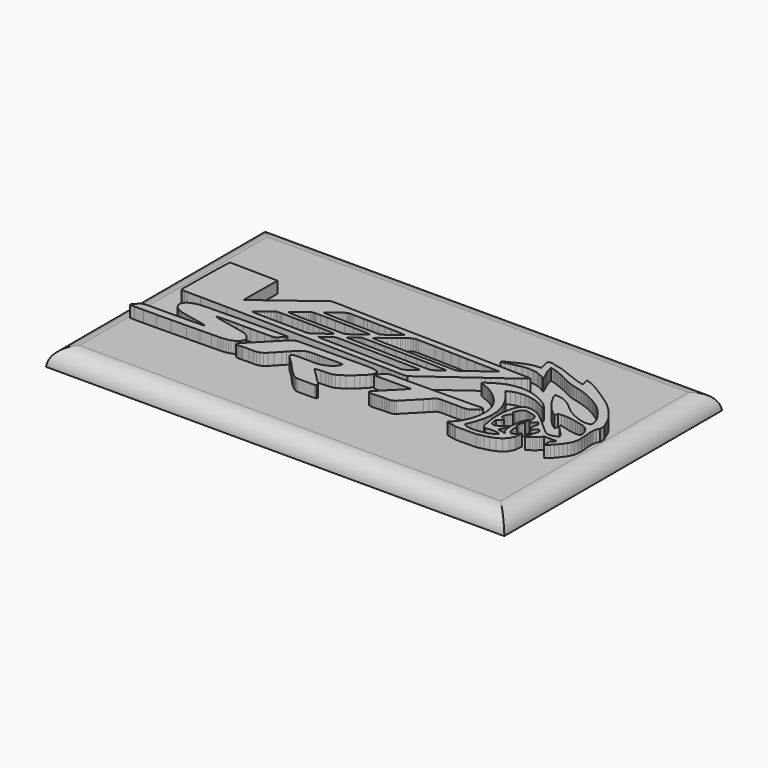
from build123d import *

# Parameters (mm, degrees)
F0_W        = 125.6636679173
F0_H        = 74.59346205
F1_DEPTH    = 4.7625
F3_DEPTH    = 3.175
F4_T1_DEPTH = 151.0140100007
F4_T3_DEPTH = 99.9438041335


# Not quite as in the source:
# - a fillet or chamfer that OpenCascade refuses, or shapes differently, is made with other operations: its cross-section is extruded or revolved along the edge and cut away or added


with BuildPart() as f1:
    # F0 (on Top) → F1 (new body)
    with BuildSketch(Plane.XY):
        Rectangle(F0_W, F0_H)
    extrude(amount=F1_DEPTH)

    # F2 (on face) → F3 (join)
    with BuildSketch(Plane.XY.offset(4.7625)):
        Polygon((-4.9450498, -8.5601048), (-4.421759, -8.639302), (-4.5465492, -9.1872054), (-4.8525684, -9.7208086), (-5.3076602, -10.224897), (-5.8802524, -10.6841036), (-6.5382648, -11.0831122), (-7.2498712, -11.4066066), (-7.9832708, -11.6391944), (-8.7064596, -11.7656102), (-9.5160592, -11.8009924), (-10.570972, -11.7964966), (-11.7620542, -11.7747034), (-12.9804668, -11.7577108), (-14.1171676, -11.7679978), (-15.0630636, -11.8277894), (-15.7091634, -11.95959), (-15.9465518, -12.1857008), (-15.8717742, -12.453112), (-15.6735526, -12.76731), (-15.3829512, -13.113512), (-15.0311612, -13.476605), (-14.2674594, -14.193901), (-13.6305544, -14.7994116), (-13.1164584, -15.3579068), (-12.4780548, -16.0731962), (-11.7503702, -16.876903), (-10.968355, -17.700498), (-10.1670612, -18.4758076), (-9.3814646, -19.134201), (-8.6465664, -19.6075046), (-7.9972662, -19.8271892), (-3.2755586, -19.8046086), (-2.797556, -19.6833998), (-2.6407618, -19.4626992), (-2.745867, -19.1551052), (-3.053461, -18.773394), (-3.504057, -18.330291), (-4.0383714, -17.8386994), (-4.5968666, -17.3112938), (-5.120259, -16.760698), (-5.4525672, -16.3987988), (-5.8057542, -16.0437068), (-6.1711586, -15.6935932), (-6.539865, -15.3470102), (-6.9028564, -15.0022052), (-7.2514714, -14.6572986), (-7.5766676, -14.3107918), (-7.869555, -13.9610084), (-6.2843664, -13.790803), (-5.0888646, -13.7265918), (-4.1617646, -13.6871964), (-3.381756, -13.5911082), (-2.6275538, -13.3571996), (-1.7779492, -12.9041906), (-0.711454, -12.1509028), (0.6931406, -11.0159038), (1.6305276, -10.2006908), (2.5060402, -9.348597), (3.211449, -8.5052916), (3.6384484, -7.716901), (3.6787328, -7.0292976), (3.2240474, -6.4884046), (2.1661374, -6.140196), (0.3966464, -6.030595), (-16.7135556, -6.2076076), (-17.6600612, -6.2193932), (-18.3821578, -6.2480952), (-18.9333632, -6.3112904), (-19.3670682, -6.4268096), (-19.7366636, -6.612509), (-20.0956672, -6.8859908), (-20.4974698, -7.265289), (-20.9954622, -7.7680058), (-28.045664, -14.961108), (-28.1941524, -15.2684988), (-28.1600656, -15.4747976), (-27.9811734, -15.5981908), (-27.6953726, -15.657195), (-27.3407632, -15.6701998), (-26.9550642, -15.6555948), (-26.576274, -15.6316934), (-26.242264, -15.6170122), (-24.5495572, -15.6137102), (-23.3030522, -15.6145992), (-22.3775524, -15.5568904), (-21.6474548, -15.3779982), (-20.9874612, -15.0153116), (-20.2721718, -14.4058894), (-19.3761614, -13.4872984), (-18.1740556, -12.196699), (-17.5040544, -11.4781076), (-16.752062, -10.6875072), (-16.366871, -10.2960932), (-15.98676, -9.923907), (-15.6206698, -9.5829882), (-15.2768554, -9.2860114), (-14.7908518, -8.9778078), (-14.2279624, -8.768207), (-13.6040622, -8.639302), (-12.9347722, -8.573008), (-12.2358658, -8.551291), (-11.5231672, -8.5560916), (-10.8124498, -8.5694012), (-10.1194616, -8.5732112), (-9.5076518, -8.5608922), (-8.7845646, -8.5400896), (-7.9914496, -8.5179916), (-7.1695564, -8.5017102), (-6.3603632, -8.4984082), (-5.6050688, -8.5155024), align=None)
        Polygon((-56.7795664, -14.6026886), (-57.280556, -14.9388068), (-57.2752728, -15.4519122), (-56.0680616, -15.5184094), (-53.5015694, -15.5360116), (-49.9995698, -15.516606), (-45.9858618, -15.4722068), (-41.8842698, -15.4148028), (-38.1184658, -15.3565098), (-35.1122742, -15.3092912), (-33.2894686, -15.285212), (-32.6026526, -15.2675082), (-31.9255648, -15.2214072), (-31.2669682, -15.1413972), (-30.6357528, -15.0217886), (-30.040453, -14.8571966), (-29.4899588, -14.6420078), (-28.9930586, -14.3704056), (-28.558363, -14.0370052), (-28.1099514, -13.4955026), (-27.9135586, -12.9533904), (-27.931872, -12.4250958), (-28.12796, -11.9251984), (-28.4644592, -11.4683032), (-28.9043618, -11.068812), (-29.4103552, -10.7412028), (-29.945457, -10.5002076), (-30.9034688, -10.21969), (-32.2077588, -9.9157028), (-33.7221576, -9.5976948), (-35.310572, -9.2750132), (-36.836858, -8.9571068), (-38.1648716, -8.6536022), (-39.1583672, -8.3737958), (-39.6813532, -8.127111), (-37.7867672, -8.075295), (-35.8783636, -8.0485996), (-33.962467, -8.0388968), (-32.0455544, -8.0381094), (-30.134052, -8.0383888), (-28.2345638, -8.0315054), (-26.353262, -8.0096106), (-24.4967506, -7.9645002), (-24.1630708, -7.9471012), (-23.8976662, -7.916291), (-23.684357, -7.8685898), (-23.5072682, -7.8001114), (-23.3501692, -7.7071982), (-23.197058, -7.5861926), (-23.0320596, -7.4332084), (-22.8389688, -7.244588), (-22.525863, -6.9569076), (-22.1765622, -6.6300096), (-22.0138498, -6.4578992), (-21.8727528, -6.2830964), (-21.7635582, -6.1080904), (-21.6963498, -5.9352942), (-22.897973, -5.86359), (-25.3242572, -5.8418984), (-28.5935674, -5.8582052), (-32.3243702, -5.900293), (-36.1351576, -5.9560968), (-39.6444724, -6.0136024), (-42.4707558, -6.0605924), (-44.2323728, -6.0851034), (-46.042961, -6.2347094), (-47.4401642, -6.6143124), (-48.4317548, -7.1706994), (-49.0252512, -7.8509114), (-49.2283496, -8.60171), (-49.0487716, -9.369806), (-48.494061, -10.1022912), (-47.5718632, -10.7459018), (-47.0938606, -10.9669072), (-46.5738718, -11.1561118), (-46.02226, -11.3192052), (-45.4497694, -11.462004), (-44.8667632, -11.5901978), (-44.2839602, -11.7096032), (-43.711749, -11.8259098), (-43.1608738, -11.9449088), (-42.8145702, -12.016613), (-42.2718738, -12.123801), (-41.6006534, -12.258294), (-40.8686508, -12.4122942), (-40.1436586, -12.5778006), (-39.4932662, -12.7468884), (-38.9852662, -12.9116074), (-38.6874512, -13.0640074), (-39.391463, -13.1373118), (-40.9285694, -13.1928108), (-43.0484534, -13.2329936), (-45.5008742, -13.260705), (-48.0355656, -13.2786882), (-50.4022614, -13.2896102), (-52.3507716, -13.2961888), (-53.6307538, -13.3012942), (-54.6571678, -13.339191), (-55.3450506, -13.4348982), (-55.7820576, -13.5832088), (-56.056149, -13.7791952), (-56.2552596, -14.0178028), (-56.4670702, -14.2940024), align=None)
        Polygon((4.0287448, -8.0929988), (3.9759382, -8.375396), (13.9917424, -8.3471004), (13.730732, -8.708009), (13.242036, -9.2605098), (12.59205, -9.946005), (11.8471442, -10.7063032), (11.0737396, -11.4830098), (10.3381302, -12.2177048), (9.7068386, -12.8520952), (9.246235, -13.3277102), (8.6214458, -13.947013), (8.1675478, -14.3867124), (8.0184498, -14.5703036), (7.928737, -14.7463002), (7.903845, -14.927199), (7.9493364, -15.1253952), (8.3251294, -15.2392888), (8.7700358, -15.3008076), (9.2644468, -15.3212038), (9.7887282, -15.3118058), (10.3231442, -15.2838912), (10.8479336, -15.2487884), (11.34364, -15.2178004), (11.7905276, -15.2021032), (12.3123452, -15.2064974), (12.8007364, -15.219807), (13.2577332, -15.2258014), (13.6855454, -15.2078944), (14.0862304, -15.1499062), (14.461744, -15.035403), (14.8141436, -14.8481034), (15.145639, -14.571599), (19.1523366, -10.4836976), (20.0035414, -9.5811086), (20.5969362, -8.9512902), (21.0416394, -8.546592), (21.4469472, -8.3194906), (21.9220288, -8.2222086), (22.5761296, -8.206994), (23.5185458, -8.2263996), (24.8582434, -8.2325972), (26.4908284, -8.2333084), (27.713051, -8.2496914), (28.6145478, -8.245602), (29.285438, -8.1849976), (29.815536, -8.0315054), (30.2947324, -7.7491082), (30.8129432, -7.3015094), (31.4601352, -6.6525902), (31.8035432, -6.2350904), (31.8998346, -5.953506), (31.789751, -5.7833006), (31.514034, -5.6999886), (31.113349, -5.6791098), (30.6284376, -5.6961024), (30.1000414, -5.7264046), (29.5689274, -5.7457086), (9.5561404, -5.952109), (9.1602306, -5.9466988), (8.6710266, -5.9301126), (8.1235296, -5.9117992), (7.5532488, -5.9015884), (6.9952362, -5.9090052), (6.484747, -5.9436), (6.0570364, -6.015101), (5.7473342, -6.1331094), (5.6303418, -6.2255908), (5.4055264, -6.4247014), (5.1118262, -6.7041014), (4.7882302, -7.0370954), (4.4739306, -7.3972928), (4.2077386, -7.7580998), align=None)
        Polygon((30.560137, 10.9086904), (31.0405272, 11.3337086), (30.5953414, 11.4064034), (30.0228508, 11.457305), (29.3624508, 11.4908076), (28.6534352, 11.5112038), (27.9352502, 11.5229894), (27.2471388, 11.5305078), (26.6284456, 11.538204), (26.1185406, 11.5502944), (20.4317346, 11.729212), (14.707743, 11.868912), (8.9595452, 11.9830088), (3.1997396, 12.0850914), (-2.5587706, 12.1885964), (-8.3031584, 12.307189), (-14.020673, 12.4544074), (-19.698462, 12.6437898), (-20.1191622, 12.6592076), (-20.7461612, 12.6799086), (-21.5059514, 12.7007874), (-22.324949, 12.7169926), (-23.129367, 12.7235966), (-23.8456724, 12.715494), (-24.4001544, 12.687808), (-24.719153, 12.6355094), (-36.6615726, 3.6841938), (-38.1194564, 2.590292), (-38.4727704, 2.3146004), (-38.8779512, 1.992503), (-39.089457, 1.843405), (-39.3012676, 1.7179036), (-39.5091666, 1.6279114), (-39.708963, 1.5849092), (-39.5792706, 12.9772918), (-52.8131532, 13.2104892), (-52.8919694, 11.9055896), (-52.9518626, 10.2175056), (-52.9962618, 8.2658966), (-53.0283674, 6.170803), (-53.0515576, 4.0520112), (-53.0691598, 2.0294092), (-53.0844506, 0.2227072), (-53.100859, -1.2480036), (-53.1241508, -1.9560032), (-53.148357, -2.4705056), (-53.1395686, -2.822194), (-53.0638512, -3.0420056), (-52.8874736, -3.1606998), (-52.5764506, -3.208909), (-52.0969494, -3.2174942), (-51.4152642, -3.2171894), (-47.769653, -3.2425894), (-40.5159718, -3.3504124), (2.7827478, -4.1852088), (3.3846262, -4.2026078), (4.2793412, -4.2317924), (5.3608478, -4.2646092), (6.523228, -4.2928032), (7.6607416, -4.3081956), (8.6674452, -4.3027092), (9.4374462, -4.2681906), (9.8648266, -4.1963086), (22.663531, 5.1201066), (23.2379266, 5.531104), (24.2443508, 6.2514988), (25.5343406, 7.1790052), (26.959433, 8.2109056), (28.371038, 9.2447872), (29.620845, 10.178288), align=None)
        Polygon((-33.6645504, -1.7394936), (-34.9256604, -1.6497046), (-34.7867732, -1.4484096), (-34.4552524, -1.1359896), (-33.9890608, -0.7499096), (-33.4457548, -0.3271012), (-32.8831702, 0.0950976), (-32.358965, 0.4796028), (-31.9308734, 0.7892034), (-31.656655, 0.9866884), (-31.3305698, 1.2276074), (-31.085155, 1.4076934), (-30.8845712, 1.5357094), (-30.6929536, 1.620393), (-30.4744628, 1.6705072), (-30.1931578, 1.6948912), (-29.8131738, 1.702308), (-29.2986714, 1.7013936), (-26.3820656, 1.6632936), (-24.9446542, 1.640205), (-23.48865, 1.6244062), (-22.0210634, 1.610487), (-20.5483714, 1.5930118), (-19.0774574, 1.5664942), (-17.6150524, 1.525397), (-16.167862, 1.4642084), (-14.742668, 1.3775944), (-14.8617686, 1.2030964), (-15.0341584, 1.0205974), (-15.2450546, 0.8349996), (-15.4795728, 0.651002), (-15.959963, 0.3070098), (-16.3567618, 0.0270002), (-17.125569, -0.564388), (-17.7068734, -1.0321036), (-18.1571646, -1.388999), (-18.5332624, -1.6480028), (-18.8916564, -1.8218912), (-19.2890648, -1.9235928), (-19.782155, -1.9660108), (-20.4274674, -1.961896), (-21.963761, -1.9281902), (-23.815167, -1.9059906), (-25.8636516, -1.8886932), (-27.991054, -1.8699988), (-30.079061, -1.8432018), (-32.0096642, -1.8019014), align=None, mode=Mode.SUBTRACT)
        Polygon((-16.2069526, -1.9470116), (-16.446754, -1.8266918), (-15.8980632, -1.4556994), (-15.4226514, -1.0815066), (-14.99235, -0.7209028), (-14.5788634, -0.3904996), (-14.1540738, -0.1070102), (-13.689457, 0.1131062), (-13.157073, 0.2530094), (-12.5284738, 0.2960116), (10.0730304, -0.201295), (9.9530408, -0.3319018), (9.6614488, -0.604393), (9.2428314, -0.9705086), (8.7416386, -1.3818108), (8.202549, -1.7899126), (7.6699364, -2.1463), (7.1885302, -2.4026114), (6.8028312, -2.5105106), (6.3747396, -2.5166066), (5.897245, -2.5015952), (5.4142386, -2.4790908), (4.970145, -2.4625046), (-9.3823536, -2.1745956), (-13.0148584, -2.0992084), (-13.3876542, -2.0981924), (-13.8466576, -2.1028914), (-14.3567658, -2.1058124), (-14.8828506, -2.0992084), (-15.3899616, -2.0756118), (-15.8429706, -2.0274026), align=None, mode=Mode.SUBTRACT)
        Polygon((-27.8380698, 2.9001974), (-28.6586676, 3.009011), (-28.4420564, 3.288411), (-28.0859738, 3.628898), (-27.6302724, 4.0091106), (-27.1145508, 4.4076112), (-26.5787632, 4.8032924), (-26.062559, 5.1747928), (-25.6055622, 5.5007002), (-25.2476508, 5.759704), (-25.031065, 5.9200034), (-24.8581672, 6.0411868), (-24.708358, 6.1287914), (-24.561165, 6.188202), (-24.3959634, 6.224905), (-24.192357, 6.2443868), (-23.9296702, 6.2521084), (-23.5873544, 6.2534038), (-22.4404682, 6.2504066), (-20.5767686, 6.23951), (-18.2504588, 6.218301), (-15.7157674, 6.1842904), (-13.2267706, 6.1348112), (-11.0377732, 6.0673996), (-9.4027498, 5.9794902), (-8.5759544, 5.8685938), (-8.757158, 5.6912002), (-8.9485724, 5.5221886), (-9.1484704, 5.3598064), (-9.3551502, 5.2020978), (-9.7821496, 4.892802), (-10.2160578, 4.5793914), (-10.9113574, 4.047998), (-11.4582702, 3.612388), (-11.9033544, 3.265805), (-12.2930666, 3.0012894), (-12.6740666, 2.8120086), (-13.0928618, 2.6907998), (-13.595858, 2.6310082), (-14.2298674, 2.6254964), (-15.6094684, 2.6502106), (-17.5122586, 2.67081), (-19.7371716, 2.6926032), (-22.0831664, 2.721102), (-24.3492528, 2.7615896), (-26.3345676, 2.8195016), align=None, mode=Mode.SUBTRACT)
        Polygon((-21.166963, 7.4673968), (-22.5784664, 7.5470004), (-22.4086674, 7.7727048), (-22.072473, 8.086598), (-21.6188544, 8.4589112), (-21.0971638, 8.8597994), (-20.5562708, 9.2594938), (-20.045553, 9.6280986), (-19.6140578, 9.9357942), (-19.3109596, 10.1528118), (-18.9929516, 10.3791004), (-18.737453, 10.5426002), (-18.5156602, 10.6527092), (-18.2988712, 10.7189016), (-18.0580538, 10.7506008), (-17.7644552, 10.7572048), (-17.3892718, 10.7481878), (-16.903573, 10.7329986), (-14.109065, 10.6643932), (-13.097764, 10.6466894), (-11.6615718, 10.6258106), (-9.9529646, 10.5999026), (-8.1238598, 10.5671874), (-6.3266574, 10.5259886), (-4.7135542, 10.4745028), (-3.4367724, 10.4109012), (-2.648458, 10.3335074), (-2.7795728, 10.1570028), (-3.1052516, 9.8624898), (-3.5671506, 9.4886018), (-4.1071546, 9.073896), (-4.666869, 8.6570058), (-5.18795, 8.2767932), (-5.6121554, 7.97179), (-5.8812684, 7.7806042), (-6.228969, 7.5359006), (-6.4874648, 7.3648062), (-6.6944494, 7.2554084), (-6.8875656, 7.1954898), (-7.1045578, 7.1732902), (-7.3830688, 7.1764906), (-7.7608684, 7.1933054), (-8.275574, 7.2115934), (-11.1920528, 7.2487028), (-12.6103634, 7.2760078), (-14.0348716, 7.296912), (-15.463266, 7.3159874), (-16.8930574, 7.3380092), (-18.3218582, 7.3674986), (-19.7472554, 7.4091038), align=None, mode=Mode.SUBTRACT)
        Polygon((-8.7423498, 1.5164054), (-11.5343686, 1.5914878), (-11.4738658, 1.7419066), (-11.4031522, 1.844294), (-11.2963706, 1.943989), (-11.1276638, 2.0862036), (-10.6380534, 2.450592), (-10.1958648, 2.7770074), (-9.8806508, 3.040888), (-9.6477582, 3.2476948), (-9.4526608, 3.402711), (-9.250553, 3.5113976), (-8.9968578, 3.5790886), (-8.647049, 3.6113974), (-8.1564734, 3.6135056), (-5.3978556, 3.5666934), (-2.5350724, 3.5265106), (0.3919474, 3.4869882), (3.343529, 3.4424112), (6.2798452, 3.3869884), (9.1608402, 3.3149032), (11.9469408, 3.220212), (14.5982436, 3.0973014), (14.46784, 2.9187902), (14.2046452, 2.6480008), (13.834745, 2.3208996), (13.3838442, 1.973199), (12.877927, 1.6407892), (12.3429268, 1.359408), (11.8047262, 1.1648948), (11.2891316, 1.093089), (8.5328506, 1.1131042), (5.703951, 1.1535918), (2.8248356, 1.2104116), (-0.0818642, 1.2792964), (-2.9935678, 1.356106), (-5.887974, 1.436497), align=None, mode=Mode.SUBTRACT)
        Polygon((-6.0683648, 4.7966884), (-7.1581518, 4.866894), (-6.9075554, 5.166487), (-6.3484506, 5.6504078), (-5.5785512, 6.2552072), (-4.695952, 6.91769), (-3.79857, 7.5747118), (-2.9842714, 8.1626964), (-2.3509732, 8.6187026), (-1.9966686, 8.879205), (-1.4768576, 9.2888054), (-1.0537698, 9.6216978), (-0.6962648, 9.8838004), (-0.3729736, 10.0812092), (-0.0526542, 10.2198932), (0.2958338, 10.3059992), (0.703834, 10.345293), (1.2026392, 10.3439976), (5.8098436, 10.2296976), (8.0340454, 10.1691948), (10.2696264, 10.1009958), (12.512548, 10.0293932), (14.7587462, 9.9586034), (17.0042332, 9.8929952), (19.244945, 9.836912), (21.4767414, 9.7943924), (23.6956346, 9.7700084), (23.5504482, 9.5602044), (23.2856278, 9.3020896), (22.9365302, 9.01319), (22.5382328, 8.7111078), (21.734526, 8.1372964), (21.1558378, 7.721092), (20.476845, 7.2081898), (19.816826, 6.7336924), (19.1565276, 6.2676024), (18.4769506, 5.779897), (17.93875, 5.3738018), (17.518634, 5.0435002), (17.177639, 4.7833026), (16.8769284, 4.5870876), (16.5777418, 4.449191), (16.2410394, 4.3636946), (15.8280354, 4.324604), (15.2998424, 4.3262042), (1.81483, 4.6383956), (0.7114286, 4.6602904), (-0.4115562, 4.6742096), (-1.5467584, 4.684903), (-2.6872692, 4.6975014), (-3.8257734, 4.716907), (-4.955159, 4.7483014), align=None, mode=Mode.SUBTRACT)
        Polygon((32.380047, -16.0050988), (32.5152258, -16.0567116), (38.3087372, -15.9968946), (38.9413496, -15.798292), (39.9464276, -15.5827984), (41.1772354, -15.2748996), (42.4866308, -14.7992084), (43.7278272, -14.080109), (44.7537332, -13.0421126), (45.4175368, -11.6099082), (45.5721466, -9.7079054), (45.3336406, -9.858502), (45.1495414, -10.0535994), (44.9928488, -10.2733094), (44.836334, -10.4974898), (44.6528444, -10.7061), (44.415329, -10.8789978), (44.0965336, -10.9961934), (43.669331, -11.0375954), (43.3635404, -10.7725972), (43.1206402, -10.4801924), (42.9409352, -10.1603048), (42.825035, -9.81329), (42.7732444, -9.4393004), (42.7859444, -9.0384122), (42.863643, -8.6107016), (43.0067466, -8.1564988), (42.5176442, -7.7380084), (42.394251, -7.4679048), (42.3420286, -7.1595996), (42.3526458, -6.8301108), (42.4176444, -6.4965072), (42.528744, -6.1762132), (42.6776388, -5.886196), (42.8558452, -5.6438038), (43.0552352, -5.4660038), (42.9651414, -5.3001926), (42.8605442, -5.1416966), (42.8132494, -5.0510948), (42.7749462, -4.9452022), (42.7497494, -4.818507), (42.74185, -4.665091), (42.7694344, -4.4936918), (42.8285402, -4.3035982), (42.8900336, -4.0799004), (42.92473, -3.8074092), (42.4467274, -4.3829986), (42.0885366, -5.0809906), (41.8371274, -5.87121), (41.6794442, -6.7233038), (41.6024314, -7.6070968), (41.5930334, -8.4923122), (41.6382454, -9.3486986), (41.7250372, -10.1460046), (41.7805362, -10.4851962), (41.8460428, -10.7548934), (41.9248336, -10.971403), (42.0203376, -11.1508032), (42.1360346, -11.3094008), (42.2751504, -11.4632994), (42.4411394, -11.6287042), (42.6374306, -11.821795), (40.4531322, -11.4625882), (40.541829, -11.0999016), (40.692451, -10.783189), (40.8776424, -10.491089), (41.069641, -10.2023926), (41.2411418, -9.8956114), (41.364535, -9.5496126), (41.4122362, -9.1429078), (41.3567372, -8.6542118), (40.6959308, -9.1988894), (40.0021298, -9.712706), (39.3145264, -10.1269038), (38.6724398, -10.3726996), (38.1150368, -10.3813102), (37.6814334, -10.0840032), (37.4109488, -9.4119954), (37.3426482, -8.2965036), (37.7731274, -7.9920084), (38.1262382, -7.7346048), (38.2745488, -7.6056998), (38.404546, -7.467092), (38.516433, -7.3116948), (38.6106416, -7.1322946), (38.4561334, -7.0092062), (38.3047494, -6.906895), (38.1553466, -6.8188078), (38.0066296, -6.7383914), (37.706935, -6.5746122), (37.3959374, -6.3631064), (37.3745506, -5.9075066), (37.4319292, -5.5110126), (37.5530364, -5.1656996), (37.7222258, -4.8633888), (37.924232, -4.5962062), (38.1437388, -4.3558968), (38.3652268, -4.134612), (38.573329, -3.9241984), (38.4922268, -3.7995098), (38.424231, -3.713099), (38.362636, -3.652901), (38.3007362, -3.6068), (38.1489458, -3.5081972), (37.9149356, -3.3198054), (37.948235, -3.078099), (38.0165356, -2.8228036), (38.1130302, -2.5614884), (38.230937, -2.3015956), (38.3633472, -2.0505928), (38.5034282, -1.8162016), (38.644449, -1.6056102), (38.77945, -1.426591), (38.9928354, -1.2187936), (39.237031, -1.0772902), (39.5079474, -0.993394), (39.8017492, -0.9582912), (40.1145502, -0.963295), (40.4422356, -0.9995916), (40.7810462, -1.0584942), (41.1269434, -1.131189), (42.0337488, -1.3830046), (42.6194474, -1.6639032), (42.9564292, -1.9832066), (43.1172366, -2.3499064), (43.1744374, -2.7734006), (43.200447, -3.2629094), (43.2677316, -3.8276022), (43.4488336, -4.4766992), (43.6525416, -4.4653962), (43.840146, -4.4392088), (44.0125358, -4.3967908), (44.170727, -4.336796), (44.3159388, -4.2575988), (44.4489332, -4.1579038), (44.5709294, -4.0362886), (44.6828418, -3.8913054), (44.7373502, -3.7960046), (44.9654422, -3.3866074), (45.2382382, -3.6563046), (45.5012298, -3.9067994), (45.6059286, -4.0402002), (45.68063, -4.1870122), (45.7161392, -4.3534076), (45.7030328, -4.5455078), (45.659929, -4.6908974), (45.6094338, -4.7706026), (45.556932, -4.8283114), (45.5081386, -4.9077118), (45.4682352, -5.0523902), (45.4430384, -5.3062124), (45.437933, -5.7126124), (45.4583292, -6.3155068), (45.5345292, -6.8525898), (45.6861418, -7.1018908), (45.9004416, -7.1242936), (46.1649318, -6.9809106), (46.4670394, -6.7324986), (46.7941406, -6.4401954), (47.1337386, -6.1648086), (47.4733366, -5.9673998), (47.7289368, -6.3797942), (47.8908364, -6.6385948), (47.9717354, -6.796913), (47.9842322, -6.9077078), (47.940849, -7.0241922), (47.8543366, -7.199503), (47.737141, -7.4865992), (47.6020384, -7.9385922), (47.4587316, -8.4944966), (47.2793314, -9.2257118), (47.1968322, -9.5997014), (47.1301318, -9.9485958), (47.087536, -10.2495096), (47.0773506, -10.479405), (47.5445328, -10.1537008), (47.9825304, -9.859391), (48.3940358, -9.5790004), (48.7819446, -9.295003), (49.1489492, -8.9898982), (49.4979452, -8.6460076), (49.8316504, -8.2460084), (50.1528334, -7.7721968), (53.6081478, -7.780909), (53.464333, -7.9891128), (53.3238456, -8.1329022), (53.1886414, -8.236204), (53.0606508, -8.322691), (52.9416264, -8.4161122), (52.833651, -8.539988), (52.7384264, -8.718296), (52.658137, -8.974709), (52.6004282, -9.3572076), (52.566951, -9.8486976), (52.5554448, -10.3528114), (52.5635474, -10.7725972), (53.048027, -10.4401112), (53.6110434, -9.9490022), (54.2173414, -9.3347032), (54.8316404, -8.6322916), (55.4185328, -7.8774036), (55.9430428, -7.1051928), (56.3696358, -6.3509906), (56.6631328, -5.6502046), (56.8864496, -4.5807122), (56.930036, -3.4619946), (56.8630308, -2.3264114), (56.7542426, -1.2057888), (56.6726324, -0.1324102), (56.6872374, 0.861695), (56.8668408, 1.7444974), (57.2805306, 2.4838914), (57.2648334, 4.0092884), (57.0800484, 4.302506), (56.9176408, 4.6187106), (56.7709304, 4.9520094), (56.6333386, 5.2965096), (56.4983376, 5.6464962), (56.3592472, 5.9960002), (56.2095396, 6.339205), (56.042433, 6.670294), (55.5521368, 7.481697), (54.9711372, 8.3111086), (54.3181286, 9.1416886), (53.612034, 9.9566984), (52.8714462, 10.738993), (52.1150342, 11.4720116), (51.3616448, 12.1387108), (50.6298454, 12.7221996), (49.7745258, 13.345795), (48.6617264, 14.1215872), (47.3709492, 14.9833076), (45.9816454, 15.8645098), (44.5732408, 16.6987982), (43.225339, 17.4198026), (42.0172388, 17.9612036), (41.0286454, 18.256504), (41.4862264, 16.2491928), (40.6892506, 16.3930076), (39.7776446, 16.6537894), (38.7764274, 17.0030902), (37.7103386, 17.412589), (36.6041432, 17.8540918), (35.4827332, 18.299303), (34.3709498, 18.7198), (33.293431, 19.0873888), (32.6046338, 19.2600072), (31.8636396, 19.4080892), (31.4962286, 19.4883024), (31.1430416, 19.5808092), (30.8131464, 19.6917056), (30.5156362, 19.8271892), (29.1086286, 19.8127112), (29.7795442, 16.6630096), (28.7129474, 16.6206932), (27.6830282, 16.4603938), (26.6867386, 16.2025076), (25.720929, 15.8671006), (24.7823482, 15.4745944), (23.8679482, 15.0450042), (22.9745286, 14.5988024), (22.0989398, 14.1561058), (21.741638, 13.9888976), (21.5242394, 13.8723878), (21.4470488, 13.8027918), (21.3798404, 13.709396), (21.3142322, 13.5802116), (21.2418422, 13.4029958), (22.2923354, 13.6463024), (23.493349, 13.9649962), (24.813133, 14.2924022), (26.2203438, 14.561693), (27.6830282, 14.7062952), (29.169741, 14.6594068), (30.6488338, 14.3544036), (32.0885312, 13.7244074), (32.4177406, 13.5071104), (32.6742298, 13.305409), (32.794448, 13.212191), (32.9196446, 13.1250944), (33.0576428, 13.044805), (33.2160372, 12.9721102), (33.034351, 13.5404098), (32.7860406, 14.1379956), (32.4983348, 14.7590002), (32.198437, 15.397607), (31.9135506, 16.0477962), (31.6709298, 16.7035988), (31.4977272, 17.3590966), (31.4211462, 18.0083968), (32.172148, 17.842992), (33.0303378, 17.5791114), (33.9554312, 17.241393), (34.9072454, 16.8546018), (35.84575, 16.4432996), (36.7305336, 16.032099), (37.5217436, 15.6457904), (38.1789432, 15.3089102), (39.0088374, 14.9171914), (39.803451, 14.6214084), (40.589835, 14.3861028), (41.3955484, 14.175994), (42.2477438, 13.955903), (43.1739294, 13.6903968), (44.201334, 13.3441948), (45.3572372, 12.8820926), (46.1988408, 12.4989082), (47.0186258, 12.0869964), (47.8116392, 11.648694), (48.572928, 11.186287), (49.2974376, 10.7020106), (49.9802404, 10.1978968), (50.616231, 9.6764094), (51.2005326, 9.1397074), (51.5914386, 8.7311992), (52.1309346, 8.1118964), (52.7474434, 7.3332086), (53.3695402, 6.4466978), (53.9254446, 5.5039006), (54.3438334, 4.5563028), (54.5531294, 3.6554918), (54.4818316, 2.8531058), (53.7156406, 2.6688034), (52.796948, 2.6853896), (51.7760458, 2.8709874), (50.7035308, 3.1935928), (49.6297458, 3.621405), (48.6052368, 4.1224962), (47.680245, 4.6648878), (46.9054434, 5.2167028), (46.2339436, 5.781802), (45.558329, 6.3724028), (44.8524376, 6.958203), (44.0901328, 7.5085956), (43.2450494, 7.9931006), (42.2912286, 8.3812888), (41.2023306, 8.642604), (39.9523458, 8.74649), (40.2438362, 7.872603), (40.7395426, 6.8567046), (41.397936, 5.7629044), (42.1776398, 4.6552104), (43.0371504, 3.5976052), (43.935142, 2.6539952), (44.8300348, 1.8885916), (45.6804268, 1.3653008), (45.7222352, 1.4702028), (45.9769464, 2.2455886), (46.7322408, 2.3634954), (47.5369382, 2.3915116), (48.3737412, 2.3460964), (49.2251492, 2.2433026), (50.0740426, 2.0995894), (50.9029462, 1.931289), (51.6946388, 1.754505), (52.4317468, 1.5856966), (52.9045424, 1.4768068), (53.302027, 1.3760958), (53.6395422, 1.2721082), (53.9318454, 1.1535918), (54.1941258, 1.0091928), (54.4414456, 0.8276082), (54.68874, 0.5973064), (54.9510458, 0.3071876), (55.1143424, 0.1006094), (55.2639484, -0.117602), (55.3991272, -0.3459988), (55.5191422, -0.5832094), (55.6231298, -0.827913), (55.7105312, -1.0784078), (55.7806352, -1.3336016), (55.8325274, -1.5917926), (55.8667412, -1.9568922), (55.797831, -2.266696), (55.4626272, -2.5596088), (54.7639494, -2.6315924), (53.819933, -2.5362916), (52.7491452, -2.3273004), (51.6700262, -2.0582128), (50.7010416, -1.7825974), (49.9606316, -1.554099), (49.5672364, -1.4264132), (49.7237258, -1.9089116), (50.0714264, -2.4374094), (50.549429, -2.9948124), (51.0966466, -3.5637978), (51.6522462, -4.1271952), (52.1552424, -4.6677072), (52.5445482, -5.1681888), (52.759229, -5.6112918), (52.4404336, -5.8942986), (52.0594336, -6.1359034), (51.6314436, -6.3271908), (51.1716274, -6.4592962), (50.6951488, -6.5229994), (50.216943, -6.509512), (49.7524278, -6.4097916), (49.3165384, -6.2147958), (46.807628, -3.9910004), (46.223047, -3.4793936), (45.5646282, -2.896489), (44.8550284, -2.2773132), (44.1169298, -1.656588), (43.3732432, -1.0692892), (42.6464476, -0.5501132), (41.9594284, -0.134112), (41.334944, 0.1439926), (40.0876262, 0.4586986), (39.0789414, 0.4887976), (38.2797304, 0.255905), (37.6604276, -0.218313), (37.19195, -0.9121902), (36.844732, -1.8041112), (36.5895382, -2.8725114), (36.3971332, -4.095496), (36.3385354, -4.6242986), (36.2973366, -5.183505), (36.273232, -5.7635902), (36.2661454, -6.3550038), (36.275645, -6.9480938), (36.3016292, -7.5334114), (36.3437424, -8.1014062), (36.4017306, -8.6425024), (36.6790478, -10.5486962), (36.9611402, -11.7371114), (37.2966488, -12.3660916), (37.7343416, -12.5943106), (38.3229358, -12.5802898), (39.1111486, -12.4826014), (40.147748, -12.4596906), (41.4813496, -12.6702058), (42.006647, -12.9030984), (41.1160468, -13.5723122), (39.9287492, -14.0825982), (38.5660392, -14.4358106), (37.1493288, -14.6336004), (35.80003, -14.6779996), (34.6394278, -14.5708116), (33.7889342, -14.313789), (33.3699358, -13.9088114), (33.4973422, -13.4499096), (33.9064346, -12.5077982), (34.4349324, -11.1407956), (34.9208344, -9.4071948), (35.2020378, -7.3653904), (35.1163382, -5.0738024), (34.5017344, -2.5905968), (33.196149, 0.025908), (32.8393298, 0.544195), (32.4372478, 1.0712958), (32.0161412, 1.5904972), (31.6023498, 2.0850098), (31.2222388, 2.5378918), (30.9019448, 2.9326078), (30.6680362, 3.2521906), (30.5466496, 3.4800032), (31.5327284, 4.0202104), (32.6104504, 4.384294), (33.7532472, 4.584192), (34.9345504, 4.6317916), (36.127944, 4.5390054), (37.3067326, 4.3176952), (38.444551, 3.979799), (39.5147292, 3.537204), (40.7164286, 2.9230066), (41.0225494, 2.7311096), (41.3440372, 2.5186894), (41.5071306, 2.4156924), (41.6699446, 2.320798), (41.831133, 2.2380956), (41.9894258, 2.172208), (41.519729, 2.926588), (40.7599388, 3.675888), (39.7733266, 4.3949112), (38.6235448, 5.0583084), (37.3740426, 5.640705), (36.0882438, 6.1169042), (34.8295468, 6.4614044), (33.6616294, 6.6491104), (32.925131, 6.690106), (32.1931284, 6.680708), (31.4704476, 6.6253106), (30.7622448, 6.5279016), (30.073346, 6.3925958), (29.4088312, 6.2236096), (28.7737296, 6.025007), (28.173045, 5.8010044), (27.7058374, 5.5930038), (27.1533366, 5.3151024), (26.553033, 4.9865026), (25.9428488, 4.6265084), (25.360249, 4.2545), (24.8429272, 3.8897052), (24.4285262, 3.5514026), (24.1548412, 3.2587946), (24.8388378, 2.9447998), (25.4414274, 2.6968958), (25.9955284, 2.4788876), (26.5341354, 2.2546056), (27.0900398, 1.9876008), (27.6961346, 1.6419068), (28.3855414, 1.1812016), (29.1910262, 0.5691886), (29.666946, 0.1747012), (30.1525432, -0.2608072), (30.6374292, -0.7375906), (31.1111392, -1.255903), (31.5631322, -1.8157952), (31.983045, -2.4175974), (32.3603366, -3.0613096), (32.6845422, -3.7473128), (33.0588366, -4.8993044), (33.2615286, -6.1084968), (33.3045308, -7.3510902), (33.1997304, -8.603107), (32.95904, -9.8407982), (32.5941436, -11.0402116), (32.1171316, -12.177395), (31.5397388, -13.2285994), (31.331027, -13.5384032), (31.1091326, -13.8258042), (30.8769258, -14.095095), (30.6374292, -14.3506952), (30.148149, -14.8378926), (29.6652442, -15.3220928), (29.9319442, -15.4750008), (30.221047, -15.5849066), (30.5269392, -15.6620972), (30.8440328, -15.7168088), (31.4890404, -15.799689), (32.1108324, -15.9155892), (32.2453508, -15.9569912), align=None)
    extrude(amount=F3_DEPTH)

    # F4: fillet of radius 5.08 on 4 edges, made by hand

    # F4_s2 → F4_t1 (cut)
    with BuildSketch(Plane.YZ.offset(-75.5070050004)):
        with BuildLine():
            ThreePointArc((37.296731025, 0), (35.7047008484, 3.3851544532), (32.2266626083, 4.7625))
            Line((32.2266626083, 4.7625), (37.296731025, 4.7625))
            Line((37.296731025, 4.7625), (37.296731025, 0))
        make_face()
        with BuildLine():
            ThreePointArc((-37.296731025, 0), (-35.7047008484, 3.3851544532), (-32.2266626083, 4.7625))
            Line((-32.2266626083, 4.7625), (-37.296731025, 4.7625))
            Line((-37.296731025, 4.7625), (-37.296731025, 0))
        make_face()
    extrude(amount=F4_T1_DEPTH, mode=Mode.SUBTRACT)

    # F4_s4 → F4_t3 (cut)
    with BuildSketch(Plane.XZ.offset(-49.9719020667)):
        with BuildLine():
            ThreePointArc((-57.7617655419, 4.7625), (-61.2398037821, 3.3851544532), (-62.8318339586, 0))
            Line((-62.8318339586, 0), (-62.8318339586, 4.7625))
            Line((-62.8318339586, 4.7625), (-57.7617655419, 4.7625))
        make_face()
        with BuildLine():
            ThreePointArc((62.8318339586, 0), (61.2398037821, 3.3851544532), (57.7617655419, 4.7625))
            Line((57.7617655419, 4.7625), (62.8318339586, 4.7625))
            Line((62.8318339586, 4.7625), (62.8318339586, 0))
        make_face()
    extrude(amount=F4_T3_DEPTH, mode=Mode.SUBTRACT)


solid = f1.part
